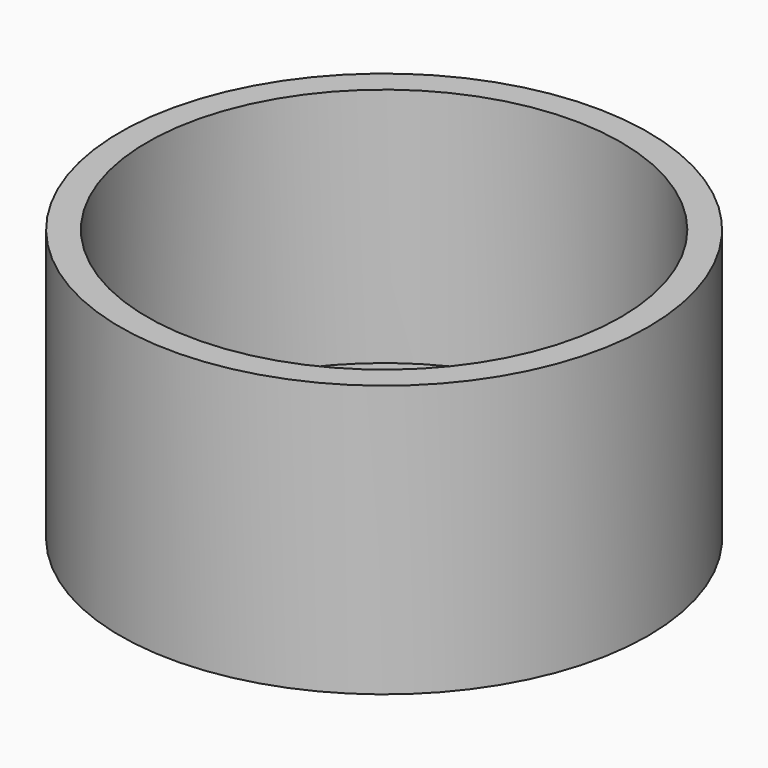
from build123d import *

# Parameters (mm, degrees)
F1_R     = 4.25
F3_DEPTH = 25
F4_SIZE  = 3.99999


# Not quite as in the source:
# - a fillet or chamfer is up to 0.001 mm smaller than in the source, because OpenCascade refuses the exact size


with BuildPart() as f2:
    # F0 (on Front) → F2 (revolve)
    with BuildSketch(Plane.XZ):
        Polygon((0, 4), (0, 0), (34, 0), (34, 35), (30.5, 35), (30.5, 4), align=None)
    revolve(axis=Axis((0, 0, 2), (0, 0, -1)))

    # F1 (on Top) → F3 (cut)
    with BuildSketch(Plane.XY):
        with Locations((-10.5, -18.1865334795)):
            Circle(F1_R)
        with Locations((-10.5, 18.1865334795)):
            Circle(F1_R)
        with Locations((21, 0)):
            Circle(F1_R)
    extrude(amount=F3_DEPTH, mode=Mode.SUBTRACT)

    # F4 (size 4 in the source; OpenCascade refuses exactly that, so slightly less here)
    f4_edges = [f2.edges().sort_by_distance(p)[0] for p in [
        (16.75, 0, 4),
        (-14.75, 18.186533, 4),
        (-14.75, -18.186533, 4),
    ]]
    chamfer(f4_edges, length=F4_SIZE)


solid = f2.part
